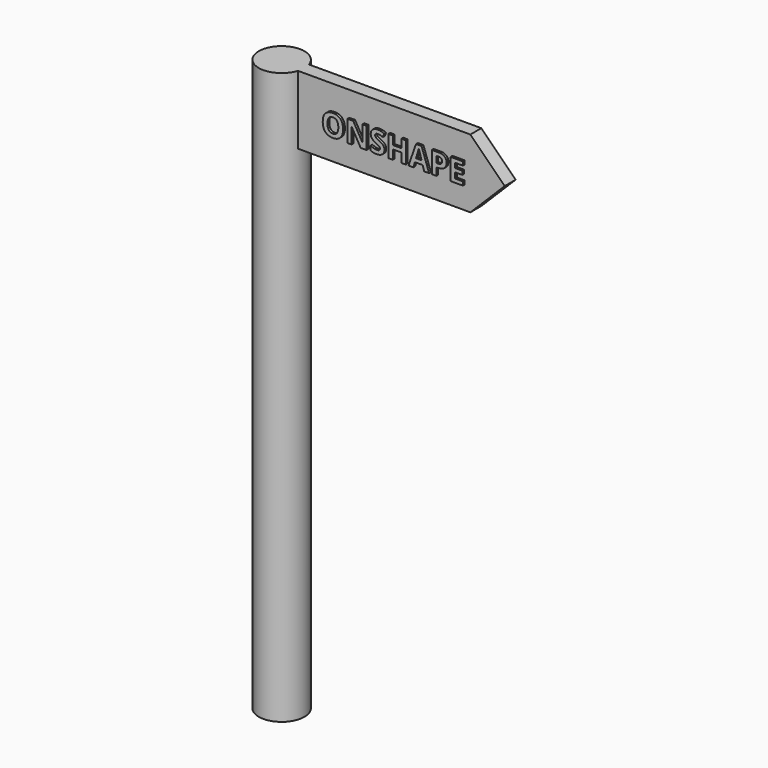
from build123d import *

# Parameters (mm, degrees)
F0_R         = 100
F1_DEPTH     = 2500
F3_DEPTH     = 30
F4_TEXT_SIZE = 130.9121979607
F5_DEPTH     = 10


# Not quite as in the source:
# - Text() gives the source's letters only with a copy of the font that has no kerning and outlines rounded to 1/6400 em; it was checked with that copy


with BuildPart() as f1:
    # F0 (on Top) → F1 (new body)
    with BuildSketch(Plane.XY):
        Circle(F0_R)
    extrude(amount=F1_DEPTH)

    # F2 (on Front) → F3 (join, symmetric)
    with BuildSketch(Plane.XZ):
        Polygon((850, 2500), (0, 2500), (0, 2200), (850, 2200), (1000, 2350), align=None)
    extrude(amount=F3_DEPTH, both=True)

    # F4 (on face) → F5 (join)
    with BuildSketch(Plane.XZ.offset(30)):
        with Locations((204.2148858309, 2298.8136768341)):
            Text('ONSHAPE', F4_TEXT_SIZE, font='Open Sans', font_style=FontStyle.BOLD, text_align=(TextAlign.LEFT, TextAlign.BOTTOM))
    extrude(amount=F5_DEPTH)


solid = f1.part
